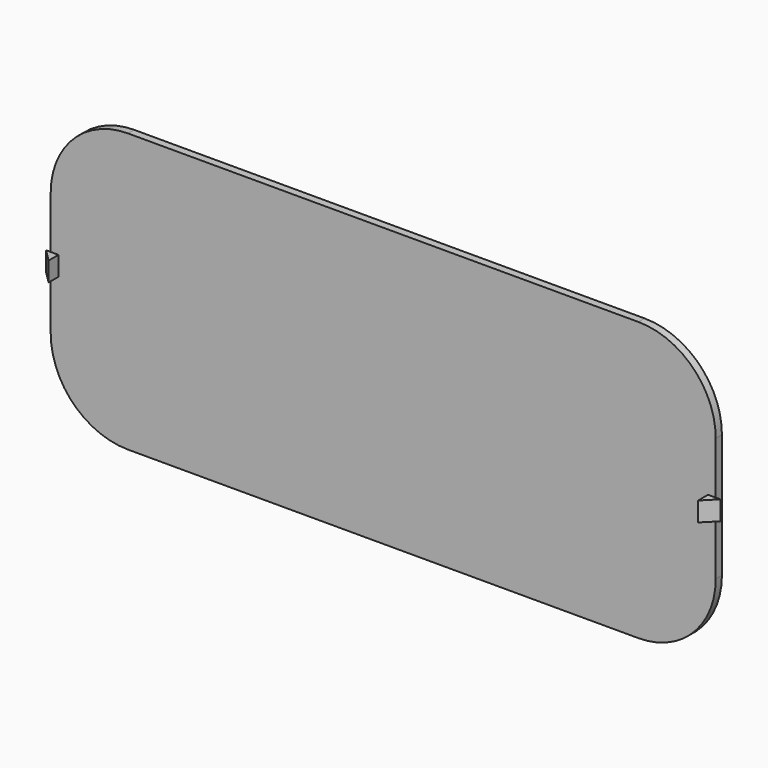
from build123d import *

# Parameters (mm, degrees)
F1_DEPTH    = 2
F0_W        = 2
F0_H        = 5
F2_DEPTH    = 6
F3_W        = 4
F3_H        = 5
F4_DEPTH    = 1.2
F5_W        = 4
F5_H        = 5
F6_DEPTH    = 1.2
F7_T1_DEPTH = 25.5734639037


# Not quite as in the source:
# - a fillet or chamfer that OpenCascade refuses, or shapes differently, is made with other operations: its cross-section is extruded or revolved along the edge and cut away or added


with BuildPart() as f1:
    # F0 (on Front) → F1 (new body)
    with BuildSketch(Plane.XZ):
        with BuildLine():
            ThreePointArc((86, 16), (80.1421356237, 30.1421356237), (66, 36))
            Line((66, 36), (-66, 36))
            ThreePointArc((-66, 36), (-80.1421356237, 30.1421356237), (-86, 16))
            Line((-86, 16), (-86, 2.5))
            Line((-86, 2.5), (-84, 2.5))
            Line((-84, 2.5), (-84, -2.5))
            Line((-84, -2.5), (-86, -2.5))
            Line((-86, -2.5), (-86, -16))
            ThreePointArc((-86, -16), (-80.1421356237, -30.1421356237), (-66, -36))
            Line((-66, -36), (66, -36))
            ThreePointArc((66, -36), (80.1421356237, -30.1421356237), (86, -16))
            Line((86, -16), (86, -2.5))
            Line((86, -2.5), (84, -2.5))
            Line((84, -2.5), (84, 2.5))
            Line((84, 2.5), (86, 2.5))
            Line((86, 2.5), (86, 16))
        make_face()
    extrude(amount=F1_DEPTH)

    # F0 (on Front) → F2 (join)
    with BuildSketch(Plane.XZ):
        with Locations((85, 0)):
            Rectangle(F0_W, F0_H)
        with Locations((-85, 0)):
            Rectangle(F0_W, F0_H)
    extrude(amount=F2_DEPTH)

    # F3 (on face) → F4 (join)
    with BuildSketch(Plane(origin=(-86, 0, 0), x_dir=(0, -1, 0), z_dir=(-1, 0, 0))):
        with Locations((4, 0)):
            Rectangle(F3_W, F3_H)
    extrude(amount=F4_DEPTH)

    # F5 (on face) → F6 (join)
    with BuildSketch(Plane.YZ.offset(86)):
        with Locations((-4, 0)):
            Rectangle(F5_W, F5_H)
    extrude(amount=F6_DEPTH)

    # F7: chamfer of 4 on 2 edges, made by hand

    # F7_s2 → F7_t1 (cut)
    with BuildSketch(Plane.XY.offset(-12.7867319519)):
        Polygon((83.2, -6), (87.2, -2), (87.2, -6), align=None)
        Polygon((-83.2, -6), (-87.2, -2), (-87.2, -6), align=None)
    extrude(amount=F7_T1_DEPTH, mode=Mode.SUBTRACT)


solid = f1.part
